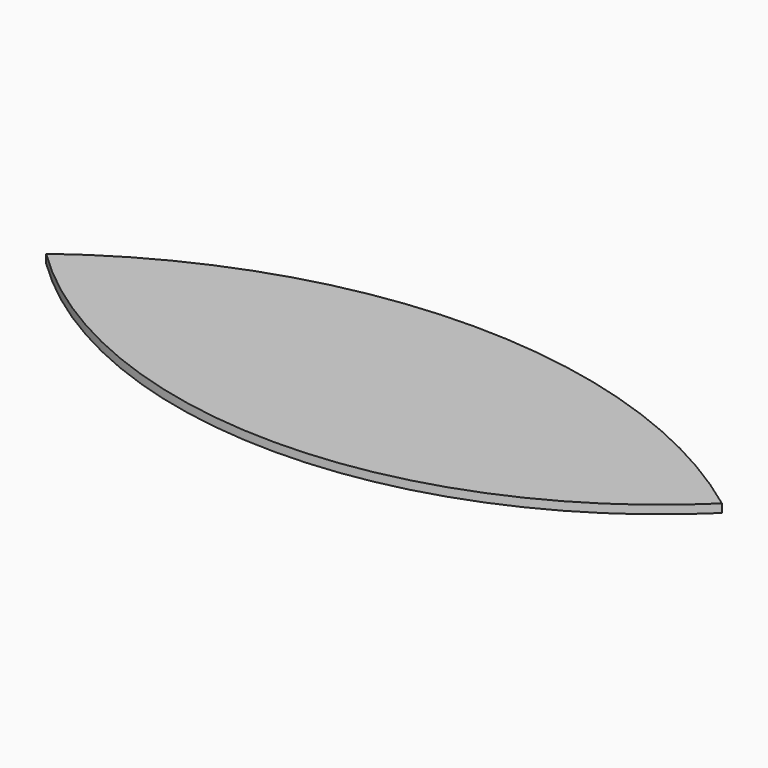
from build123d import *

# Parameters (mm, degrees)
F2_DEPTH = 0.8815038018


# Not quite as in the source:
# - the program builds the solid bodies; features that only make, move or delete a surface that nothing else refers to are left out


with BuildPart() as f2:
    # F0 (on Top) → F2 (new body)
    with BuildSketch(Plane.XY):
        with BuildLine():
            ThreePointArc((35.4751348495, 0), (0.1036971807, 11.8251612538), (-35.2677404881, 0))
            Line((-35.2677404881, 0), (35.4751348495, 0))
        make_face()
        with BuildLine():
            Line((35.4751348495, 0), (-35.2677404881, 0))
            ThreePointArc((-35.2677404881, 0), (0.1036971807, -14.3937847459), (35.4751348495, 0))
        make_face()
    extrude(amount=F2_DEPTH)


solid = f2.part
